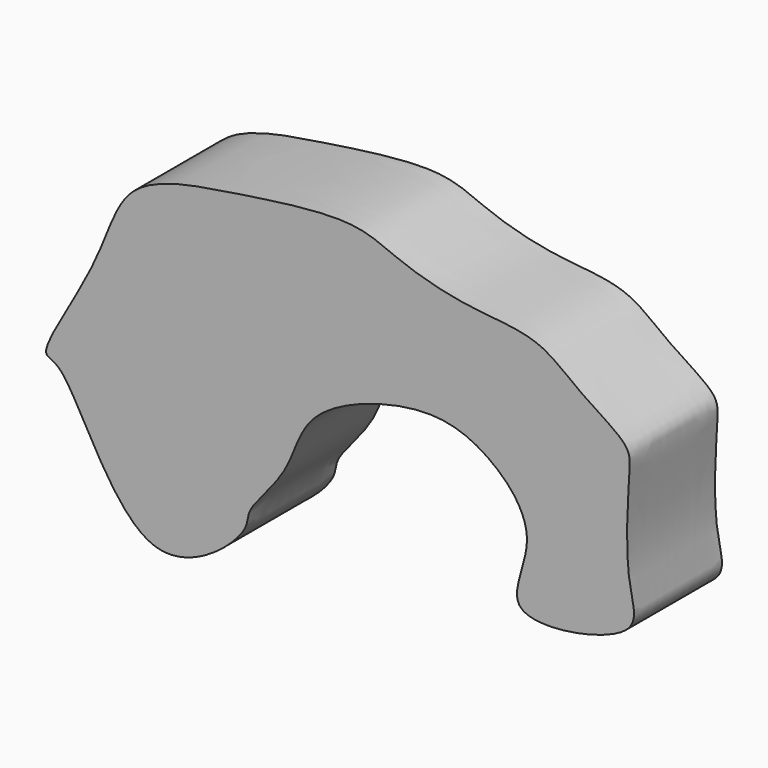
from build123d import *

# Parameters (mm, degrees)
F1_DEPTH = 20


with BuildPart() as f1:
    # F0 (on Front) → F1 (new body)
    with BuildSketch(Plane.XZ):
        with BuildLine():
            add(Edge.make_bspline(
                [(-27.7707818896, 36.6971045732), (-35.2068259317, 35.5707865733), (-48.7707734033, 33.5235680909), (-51.8118838739, 17.6688240353), (-64.7903300066, -1.2304576595), (-57.9060088757, -0.0820970655), (-45.9996826528, -34.9698414711), (-24.8213652788, -17.1691649535), (-26.242668849, -13.1109480644), (-17.465103742, -5.0071751597), (-15.853235551, 7.1688575386), (5.1388222938, 14.3910453001), (17.5755650792, 11.1459214841), (28.7399857708, -0.4968858727), (17.6829108394, -17.2884154648), (47.577110955, -11.7898307903), (42.5929647247, -2.1103929319), (43.9067861507, 15.178782936), (44.0085342563, 19.8759495054), (34.4148517734, 25.0923081147), (27.5143101021, 31.833762258), (14.3804963791, 31.9494642941), (1.9275594929, 35.377740195), (-6.3347166389, 39.9509460071), (-19.9158439897, 37.8868713222), (-27.7707818896, 36.6971045732)],
                knots=[0, 0, 0, 0, 0.0533852154, 0.1022621764, 0.1551320457, 0.1761119821, 0.2412977813, 0.2926593483, 0.3162551201, 0.3553932588, 0.3970229002, 0.450965277, 0.4948844957, 0.5399026954, 0.5808785683, 0.6342340481, 0.6689660823, 0.7194924623, 0.7445384129, 0.7826143431, 0.8205688042, 0.8638331795, 0.9071797297, 0.9436074411, 1, 1, 1, 1], degree=3))
        make_face()
    extrude(amount=F1_DEPTH)


solid = f1.part
